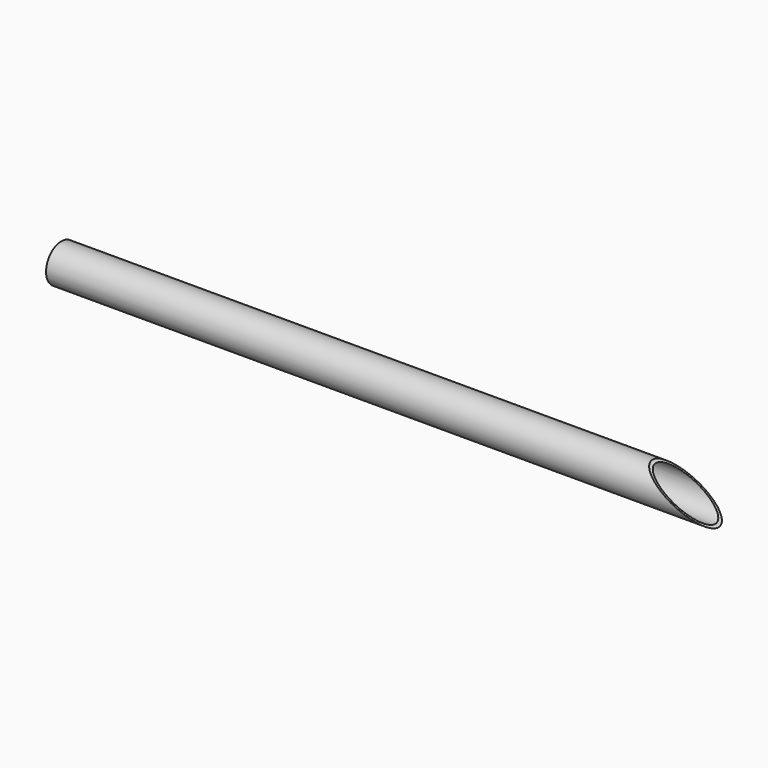
from build123d import *

# Parameters (mm, degrees)
F0_R          = 20
F0_R_2        = 18
F1_DEPTH      = 750
F3_DEPTH      = 20.001
F3_DEPTH_BACK = 20.001


with BuildPart() as f1:
    # F0 (on Right) → F1 (new body)
    with BuildSketch(Plane.YZ):
        Circle(F0_R)
        Circle(F0_R_2, mode=Mode.SUBTRACT)
    extrude(amount=F1_DEPTH)

    # F2 (on Front) → F3 (cut, two sides)
    with BuildSketch(Plane.XZ) as f3_sk:
        Polygon((620, 20), (689.2820323028, -20), (803.4400343895, -20), (803.4400343895, 20), (689.2820323028, 20), align=None)
    extrude(amount=-F3_DEPTH, mode=Mode.SUBTRACT)
    extrude(f3_sk.sketch, amount=F3_DEPTH_BACK, mode=Mode.SUBTRACT)


solid = f1.part
